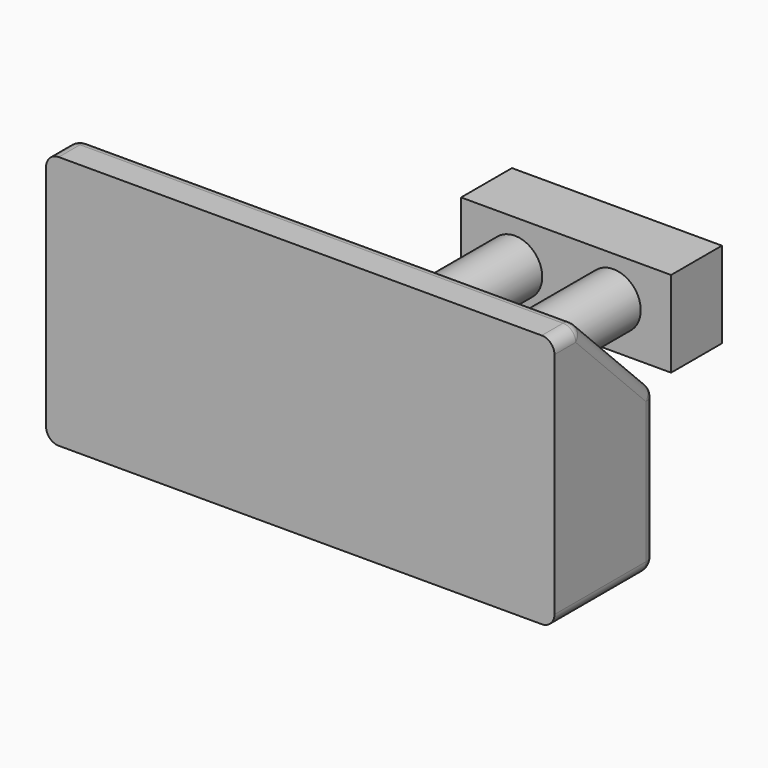
from build123d import *

# Parameters (mm, degrees)
F0_W         = 203.2
F0_H         = 101.6
F1_DEPTH     = 50.8
F2_R         = 5.08
F3_SIZE      = 38.1
F4_T1_DEPTH  = 71.12
F4_T3_DEPTH  = 58.42
F4_T6_ANGLE  = 90
F5_R         = 5.08
F6_T1_DEPTH  = 64.4773318296
F6_T3_DEPTH  = 193.04
F6_T8_DEPTH  = 5.08
F6_T14_DEPTH = 5.08
F7_T1_DEPTH  = 193.04
F7_T3_DEPTH  = 23.2957951031
F7_T8_DEPTH  = 5.08
F7_T14_DEPTH = 5.08
F8_W         = 104.7176718712
F8_H         = 41.105248034
F9_DEPTH     = 6.35
F10_R        = 10.900008085
F11_DEPTH    = 76.2
F12_W        = 83.9344151318
F12_H        = 34.3853458762
F13_DEPTH    = 25.4


# Not quite as in the source:
# - a fillet or chamfer that OpenCascade refuses, or shapes differently, is made with other operations: its cross-section is extruded or revolved along the edge and cut away or added


with BuildPart() as f1:
    # F0 (on Front) → F1 (new body)
    with BuildSketch(Plane.XZ):
        Rectangle(F0_W, F0_H)
    extrude(amount=F1_DEPTH)

    # F2
    f2_edges = [f1.edges().sort_by_distance(p)[0] for p in [
        (0, 0, -50.8),
    ]]
    fillet(f2_edges, radius=F2_R)

    # F3
    f3_edges = [f1.edges().sort_by_distance(p)[0] for p in [
        (0, 0, 50.8),
    ]]
    chamfer(f3_edges, length=F3_SIZE)

    # F4: fillet of radius 5.08 on 1 edges, made by hand

    # F4_s2 → F4_t1 (cut)
    with BuildSketch(Plane.XY.offset(-45.72)):
        with BuildLine():
            ThreePointArc((-101.6, -5.08), (-100.1121024484, -1.4878975516), (-96.52, 0))
            Line((-96.52, 0), (-101.6, 0))
            Line((-101.6, 0), (-101.6, -5.08))
        make_face()
    extrude(amount=F4_T1_DEPTH, mode=Mode.SUBTRACT)

    # F4_s4 → F4_t3 (cut)
    with BuildSketch(Plane.XZ.offset(5.08)):
        with BuildLine():
            ThreePointArc((-101.6, -45.72), (-100.1121024484, -49.3121024484), (-96.52, -50.8))
            Line((-96.52, -50.8), (-101.6, -50.8))
            Line((-101.6, -50.8), (-101.6, -45.72))
        make_face()
    extrude(amount=F4_T3_DEPTH, mode=Mode.SUBTRACT)

    # F4_s5 → F4_t6 (revolve, cut)
    with BuildSketch(Plane.XZ.offset(5.08)):
        with BuildLine():
            ThreePointArc((-101.6, -45.72), (-100.1121024484, -49.3121024484), (-96.52, -50.8))
            Line((-96.52, -50.8), (-101.6, -50.8))
            Line((-101.6, -50.8), (-101.6, -45.72))
        make_face()
    revolve(axis=Axis((-101.6, -5.08, -45.72), (1, 0, 0)), revolution_arc=F4_T6_ANGLE, mode=Mode.SUBTRACT)

    # F5
    f5_edges = [f1.edges().sort_by_distance(p)[0] for p in [
        (101.6, 0, -16.51),
    ]]
    fillet(f5_edges, radius=F5_R)

    # F6: fillet of radius 5.08 on 1 edges, made by hand

    # F6_s2 → F6_t1 (cut)
    with BuildSketch(Plane(origin=(0, -7.8378975516, 7.8378975516), x_dir=(1, 0, 0), z_dir=(0, -0.7071067812, 0.7071067812))):
        with BuildLine():
            ThreePointArc((101.6, 3.9002561211), (100.1121024484, 7.4923585695), (96.52, 8.9802561211))
            Line((96.52, 8.9802561211), (101.6, 8.9802561211))
            Line((101.6, 8.9802561211), (101.6, 3.9002561211))
        make_face()
        with BuildLine():
            ThreePointArc((-101.6, 3.9002561211), (-100.1121024484, 7.4923585695), (-96.52, 8.9802561211))
            Line((-96.52, 8.9802561211), (-101.6, 8.9802561211))
            Line((-101.6, 8.9802561211), (-101.6, 3.9002561211))
        make_face()
    extrude(amount=F6_T1_DEPTH, mode=Mode.SUBTRACT)

    # F6_s4 → F6_t3 (cut)
    with BuildSketch(Plane.YZ.offset(-96.52)):
        with BuildLine():
            ThreePointArc((0, 10.5957951031), (-0.3866919748, 12.5398269396), (-1.4878975516, 14.1878975516))
            Line((-1.4878975516, 14.1878975516), (0, 12.7))
            Line((0, 12.7), (0, 10.5957951031))
        make_face()
    extrude(amount=F6_T3_DEPTH, mode=Mode.SUBTRACT)


with BuildPart() as f6_tool6:
    # F6_s7 → F6_t8 (new body)
    with BuildSketch(Plane.YZ.offset(96.52)):
        Polygon((-5.08, 10.5957951031), (-1.4878975516, 14.1878975516), (0, 12.7), (0, 10.5957951031), align=None)
    extrude(amount=F6_T8_DEPTH)

    # F6_s9 → F6_t10 (revolve, cut)
    with BuildSketch(Plane(origin=(96.52, -5.08, 10.5957951031), x_dir=(0, -0.9238795325, -0.3826834324), z_dir=(0, -0.3826834324, 0.9238795325))):
        with BuildLine():
            ThreePointArc((0, -5.08), (5.08, 0), (0, 5.08))
            Line((0, 5.08), (0, -5.08))
        make_face()
    revolve(axis=Axis((96.52, -5.08, 10.5957951031), (1, 0, 0)), mode=Mode.SUBTRACT)


with BuildPart() as f1_1:
    add(f1.part)

    # F6_t5: cut F6_tool6
    add(f6_tool6.part, mode=Mode.SUBTRACT)


with BuildPart() as f6_tool12:
    # F6_s13 → F6_t14 (new body)
    with BuildSketch(Plane.YZ.offset(-96.52)):
        Polygon((-5.08, 10.5957951031), (-1.4878975516, 14.1878975516), (0, 12.7), (0, 10.5957951031), align=None)
    extrude(amount=-F6_T14_DEPTH)

    # F6_s15 → F6_t16 (revolve, cut)
    with BuildSketch(Plane(origin=(-96.52, -5.08, 10.5957951031), x_dir=(0, -0.9238795325, -0.3826834324), z_dir=(0, 0.3826834324, -0.9238795325))):
        with BuildLine():
            ThreePointArc((0, -5.08), (5.08, 0), (0, 5.08))
            Line((0, 5.08), (0, -5.08))
        make_face()
    revolve(axis=Axis((-96.52, -5.08, 10.5957951031), (-1, 0, 0)), mode=Mode.SUBTRACT)


with BuildPart() as f1_2:
    add(f1_1.part)

    # F6_t11: cut F6_tool12
    add(f6_tool12.part, mode=Mode.SUBTRACT)

    # F7: fillet of radius 5.08 on 3 edges, made by hand

    # F7_s2 → F7_t1 (cut)
    with BuildSketch(Plane.YZ.offset(-96.52)):
        with BuildLine():
            ThreePointArc((-40.2042048969, 50.8), (-38.2601730604, 50.4133080252), (-36.6121024484, 49.3121024484))
            Line((-36.6121024484, 49.3121024484), (-38.1, 50.8))
            Line((-38.1, 50.8), (-40.2042048969, 50.8))
        make_face()
    extrude(amount=F7_T1_DEPTH, mode=Mode.SUBTRACT)

    # F7_s4 → F7_t3 (cut)
    with BuildSketch(Plane.XZ.offset(40.2042048969)):
        with BuildLine():
            ThreePointArc((101.6, 45.72), (100.1121024484, 49.3121024484), (96.52, 50.8))
            Line((96.52, 50.8), (101.6, 50.8))
            Line((101.6, 50.8), (101.6, 45.72))
        make_face()
        with BuildLine():
            ThreePointArc((-101.6, 45.72), (-100.1121024484, 49.3121024484), (-96.52, 50.8))
            Line((-96.52, 50.8), (-101.6, 50.8))
            Line((-101.6, 50.8), (-101.6, 45.72))
        make_face()
    extrude(amount=F7_T3_DEPTH, mode=Mode.SUBTRACT)


with BuildPart() as f7_tool6:
    # F7_s7 → F7_t8 (new body)
    with BuildSketch(Plane.YZ.offset(-96.52)):
        Polygon((-40.2042048969, 45.72), (-40.2042048969, 50.8), (-38.1, 50.8), (-36.6121024484, 49.3121024484), align=None)
    extrude(amount=-F7_T8_DEPTH)

    # F7_s9 → F7_t10 (revolve, cut)
    with BuildSketch(Plane(origin=(-96.52, -40.2042048969, 45.72), x_dir=(0, -0.3826834324, -0.9238795325), z_dir=(0, 0.9238795325, -0.3826834324))):
        with BuildLine():
            ThreePointArc((0, -5.08), (5.08, 0), (0, 5.08))
            Line((0, 5.08), (0, -5.08))
        make_face()
    revolve(axis=Axis((-96.52, -40.2042048969, 45.72), (-1, 0, 0)), mode=Mode.SUBTRACT)


with BuildPart() as f1_3:
    add(f1_2.part)

    # F7_t5: cut F7_tool6
    add(f7_tool6.part, mode=Mode.SUBTRACT)


with BuildPart() as f7_tool12:
    # F7_s13 → F7_t14 (new body)
    with BuildSketch(Plane.YZ.offset(96.52)):
        Polygon((-40.2042048969, 45.72), (-40.2042048969, 50.8), (-38.1, 50.8), (-36.6121024484, 49.3121024484), align=None)
    extrude(amount=F7_T14_DEPTH)

    # F7_s15 → F7_t16 (revolve, cut)
    with BuildSketch(Plane(origin=(96.52, -40.2042048969, 45.72), x_dir=(0, -0.3826834324, -0.9238795325), z_dir=(0, -0.9238795325, 0.3826834324))):
        with BuildLine():
            ThreePointArc((0, -5.08), (5.08, 0), (0, 5.08))
            Line((0, 5.08), (0, -5.08))
        make_face()
    revolve(axis=Axis((96.52, -40.2042048969, 45.72), (1, 0, 0)), mode=Mode.SUBTRACT)


with BuildPart() as f1_4:
    add(f1_3.part)

    # F7_t11: cut F7_tool12
    add(f7_tool12.part, mode=Mode.SUBTRACT)

    # F8 (on face) → F9 (join)
    with BuildSketch(Plane(origin=(0, 0, 0), x_dir=(-1, 0, 0), z_dir=(0, 1, 0))):
        with Locations((0, -17.4928158522)):
            Rectangle(F8_W, F8_H)
    extrude(amount=F9_DEPTH)

    # F10 (on face) → F11 (join)
    with BuildSketch(Plane(origin=(0, 6.35, 0), x_dir=(-1, 0, 0), z_dir=(0, 1, 0))):
        with Locations((-18.5013078153, -16.3395497948)):
            Circle(F10_R)
        with Locations((20.8696890622, -17.3914972693)):
            Circle(F10_R)
    extrude(amount=F11_DEPTH)

    # F12 (on face) → F13 (join)
    with BuildSketch(Plane(origin=(0, 82.55, 0), x_dir=(-1, 0, 0), z_dir=(0, 1, 0))):
        with Locations((0.4271473736, -17.1926729381)):
            Rectangle(F12_W, F12_H)
    extrude(amount=F13_DEPTH)


solid = f1_4.part
